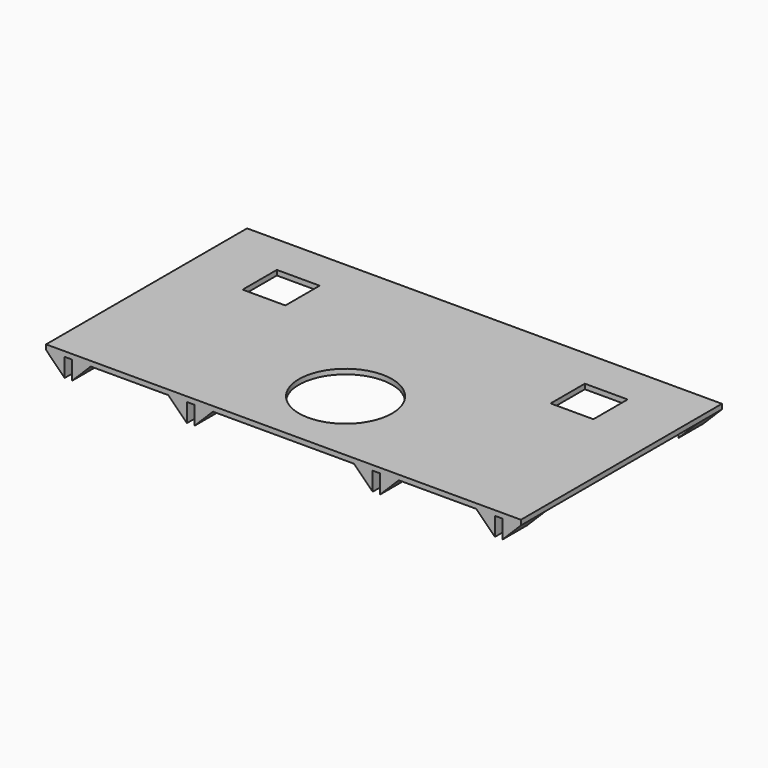
from build123d import *

# Parameters (mm, degrees)
F2_DEPTH  = 81
F3_DEPTH  = 10
F4_START  = -71
F4_DEPTH  = 10
F7_DEPTH  = 5
F9_R      = 15
F10_DEPTH = 1.6
F11_W     = 13.8
F11_H     = 13.8
F12_DEPTH = 1.6


# Not quite as in the source:
# - a feature names something its author has since deleted; it is built from what else it names


with BuildPart() as f2:
    # F1 (on offset) → F2 (new body)
    with BuildSketch(Plane.XZ.offset(40.5)):
        Polygon((76.55, 0), (76.55, 1.6), (-76.55, 1.6), (-76.55, 0), (-70.55, 0), (-68.15, 0), (-62.15, 0), (-37.15, 0), (-31.15, 0), (-28.75, 0), (-22.75, 0), (22.75, 0), (28.75, 0), (31.15, 0), (37.15, 0), (62.15, 0), (68.15, 0), (70.55, 0), align=None)
    extrude(amount=-F2_DEPTH)

    # F1 (on offset) → F3 (join)
    with BuildSketch(Plane.XZ.offset(40.5)):
        Polygon((-62.15, 0), (-68.15, 0), (-68.15, -6), align=None)
        Polygon((-31.15, 0), (-37.15, 0), (-31.15, -6), align=None)
        Polygon((-22.75, 0), (-28.75, 0), (-28.75, -6), align=None)
        Polygon((-70.55, 0), (-76.55, 0), (-70.55, -6), align=None)
    extrude(amount=-F3_DEPTH)

    # F1 (on offset) → F4 (join)
    with BuildSketch(Plane.XZ.offset(40.5).offset(F4_START)):
        Polygon((-62.15, 0), (-68.15, 0), (-68.15, -6), align=None)
        Polygon((-31.15, 0), (-37.15, 0), (-31.15, -6), align=None)
        Polygon((-22.75, 0), (-28.75, 0), (-28.75, -6), align=None)
        Polygon((-70.55, 0), (-76.55, 0), (-70.55, -6), align=None)
    extrude(amount=-F4_DEPTH)

    # F6 (on offset) → F7 (join, symmetric)
    with BuildSketch(Plane.YZ.offset(-49.65)):
        Polygon((-13.5, 0), (-13.5, -6), (-7.5, 0), align=None)
        Polygon((-17.9, -6), (-17.9, 0), (-23.9, 0), align=None)
    extrude(amount=F7_DEPTH, both=True)

    # F8: F2 across plane


with BuildPart() as f2_1:
    add(f2.part)
    add(f2.part.mirror(Plane.YZ))

    # F9 (on face) → F10 (cut)
    with BuildSketch(Plane.XY.offset(1.6)):
        with Locations((0, -15.5)):
            Circle(F9_R)
    extrude(amount=-F10_DEPTH, mode=Mode.SUBTRACT)

    # F11 (on face) → F12 (cut)
    with BuildSketch(Plane.XY.offset(1.6)):
        with Locations((-49.65, 20.6)):
            Rectangle(F11_W, F11_H)
        with Locations((49.65, 20.6)):
            Rectangle(F11_W, F11_H)
    extrude(amount=-F12_DEPTH, mode=Mode.SUBTRACT)


solid = f2_1.part
